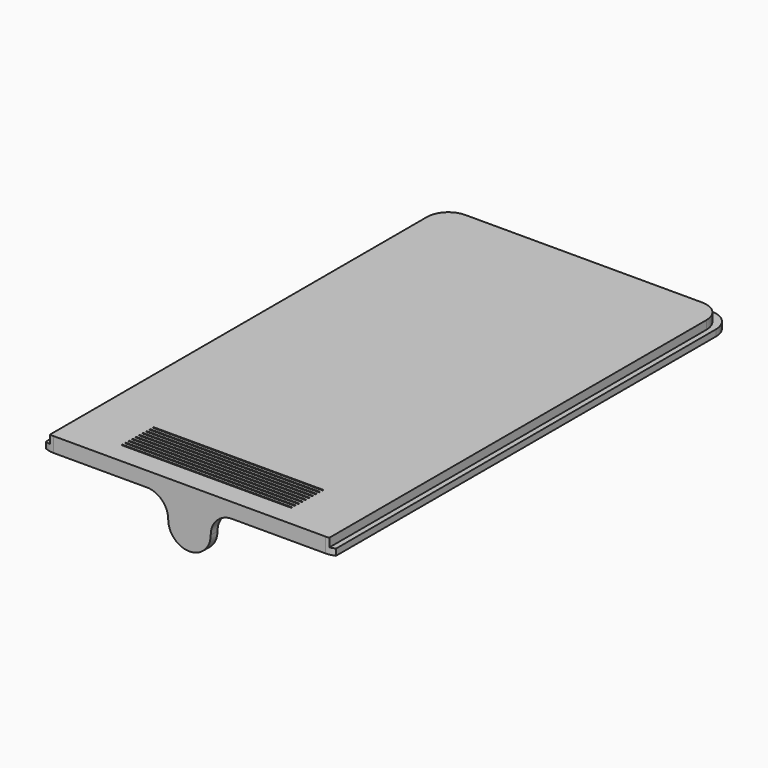
from build123d import *

# Parameters (mm, degrees)
F1_DEPTH  = 116
F2_W      = 68.25
F2_H      = 1.5
F3_DEPTH  = 1.25
F4_R      = 5
F6_DEPTH  = 25
F7_W      = 10
F7_H      = 10
F8_DEPTH  = 2
F9_R      = 4.99999
F10_W     = 5
F10_H     = 5
F11_DEPTH = 1
F12_W     = 40
F12_H     = 0.25
F13_DEPTH = 1


# Not quite as in the source:
# - a fillet or chamfer is up to 0.001 mm smaller than in the source, because OpenCascade refuses the exact size


with BuildPart() as f1:
    # F0 (on Front) → F1 (new body)
    with BuildSketch(Plane.XZ):
        Polygon((32.875, 1.5), (32.875, 3.5), (-32.875, 3.5), (-32.875, 1.5), (-34.125, 1.5), (-34.125, 0), (34.125, 0), (34.125, 1.5), align=None)
    extrude(amount=-F1_DEPTH)

    # F2 (on face) → F3 (join)
    with BuildSketch(Plane(origin=(0, 116, 0), x_dir=(-1, 0, 0), z_dir=(0, 1, 0))):
        with Locations((0, 0.75)):
            Rectangle(F2_W, F2_H)
    extrude(amount=F3_DEPTH)

    # F4
    f4_edges = [f1.edges().sort_by_distance(p)[0] for p in [
        (34.125, 117.25, 0.75),
        (-34.125, 117.25, 0.75),
        (-32.875, 116, 2.5),
        (32.875, 116, 2.5),
    ]]
    fillet(f4_edges, radius=F4_R)

    # F5 (on Top) → F6 (cut)
    with BuildSketch(Plane.XY):
        with BuildLine():
            ThreePointArc((-32, 0), (-35.5355339059, 1.4644660941), (-37, 5))
            Line((-37, 5), (-47.4459486902, 5.1317643374))
            Line((-47.4459486902, 5.1317643374), (-32.4784885049, -8.2395952195))
            Line((-32.4784885049, -8.2395952195), (-32, 0))
        make_face()
        with BuildLine():
            Line((47.8749121428, 4.8458835855), (37, 4.9999998882))
            ThreePointArc((37, 4.9999998882), (35.5355339059, 1.4644659823), (32, -1.118e-07))
            Line((32, -1.118e-07), (31.699370116, -9.054190591))
            Line((31.699370116, -9.054190591), (47.8749121428, 4.8458835855))
        make_face()
    extrude(amount=F6_DEPTH, mode=Mode.SUBTRACT)

    # F7 (on face) → F8 (join)
    with BuildSketch(Plane.XZ):
        with Locations((0, -5)):
            Rectangle(F7_W, F7_H)
    extrude(amount=-F8_DEPTH)

    # F9 (radius 5 in the source; OpenCascade refuses exactly that, so slightly less here)
    f9_edges = [f1.edges().sort_by_distance(p)[0] for p in [
        (5, 1, 0),
        (-5, 1, 0),
        (-5, 1, -10),
        (5, 1, -10),
    ]]
    fillet(f9_edges, radius=F9_R)

    # F10 (on face) → F11 (cut)
    with BuildSketch(Plane(origin=(0, 2, 0), x_dir=(-1, 0, 0), z_dir=(0, 1, 0))):
        with Locations((0, -2.5)):
            Rectangle(F10_W, F10_H)
    extrude(amount=-F11_DEPTH, mode=Mode.SUBTRACT)

    # F12 (on face) → F13 (cut)
    with BuildSketch(Plane.XY.offset(3.5)):
        with Locations((0, 5.125)):
            Rectangle(F12_W, F12_H)
        with Locations((0.0169467185, 6.1248563941)):
            Rectangle(F12_W, F12_H)
        with Locations((0.0338934371, 7.1247127881)):
            Rectangle(F12_W, F12_H)
        with Locations((0.0508401556, 8.1245691822)):
            Rectangle(F12_W, F12_H)
        with Locations((0.0677868742, 9.1244255762)):
            Rectangle(F12_W, F12_H)
        with Locations((0.0847335927, 10.1242819703)):
            Rectangle(F12_W, F12_H)
        with Locations((0.1016803113, 11.1241383643)):
            Rectangle(F12_W, F12_H)
        with Locations((0.1186270298, 12.1239947584)):
            Rectangle(F12_W, F12_H)
        with Locations((0.1355737483, 13.1238511524)):
            Rectangle(F12_W, F12_H)
        with Locations((0.1525204669, 14.1237075465)):
            Rectangle(F12_W, F12_H)
    extrude(amount=-F13_DEPTH, mode=Mode.SUBTRACT)


solid = f1.part
